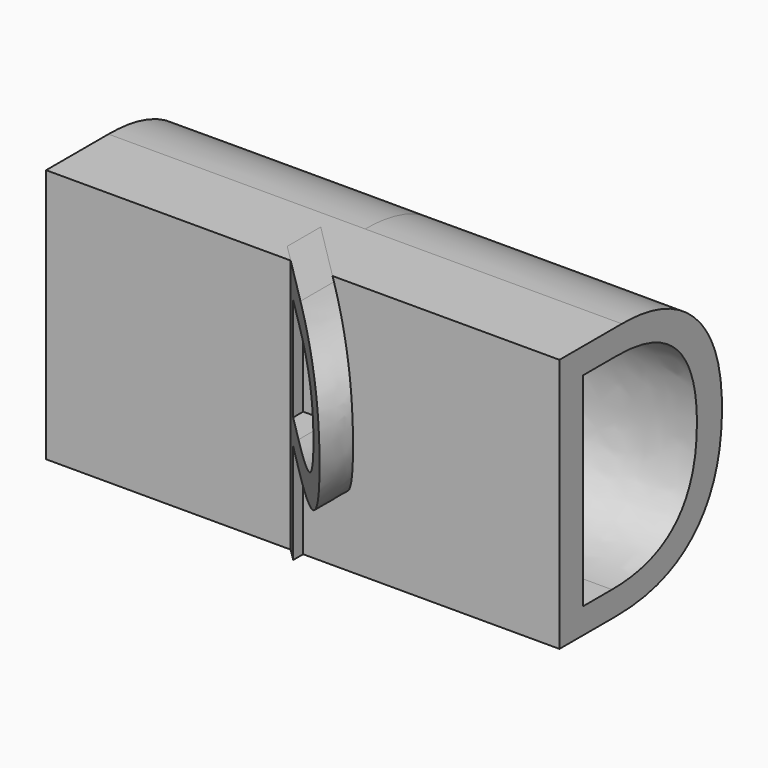
from build123d import *

# Parameters (mm, degrees)
F2_TEXT_SIZE = 138.8888888889
F5_DEPTH     = 100
F3_TEXT_SIZE = 138.8888888889
F6_DEPTH     = 100
F4_TEXT_SIZE = 138.8888888889
F7_DEPTH     = 100


# Not quite as in the source:
# - Text() gives the source's letters only with a copy of the font that has no kerning and outlines rounded to 1/6400 em; it was checked with that copy


with BuildPart() as f5:
    # F2 (on Front) → F5 (new body, symmetric)
    with BuildSketch(Plane.XZ):
        with Locations((-25, -50)):
            Text('P', F2_TEXT_SIZE, font='Open Sans', text_align=(TextAlign.LEFT, TextAlign.BOTTOM))
    extrude(amount=F5_DEPTH, both=True)


with BuildPart() as f6:
    # F3 (on face) → F6 (new body, symmetric)
    with BuildSketch(Plane(origin=(0, 0, 0), x_dir=(0.7071067812, 0.7071067812, 0), z_dir=(0.7071067812, -0.7071067812, 0))):
        with Locations((-25, -50)):
            Text('L', F3_TEXT_SIZE, font='Open Sans', text_align=(TextAlign.LEFT, TextAlign.BOTTOM))
    extrude(amount=F6_DEPTH, both=True)


with BuildPart() as f7:
    # F4 (on Right) → F7 (new body, symmetric)
    with BuildSketch(Plane.YZ):
        with Locations((-25, -50)):
            Text('D', F4_TEXT_SIZE, font='Open Sans', text_align=(TextAlign.LEFT, TextAlign.BOTTOM))
    extrude(amount=F7_DEPTH, both=True)


with BuildPart() as f5_1:
    add(f5.part)

    # F8: intersect F6
    add(f6.part, mode=Mode.INTERSECT)


solid = Compound([f7.part, f5_1.part])
